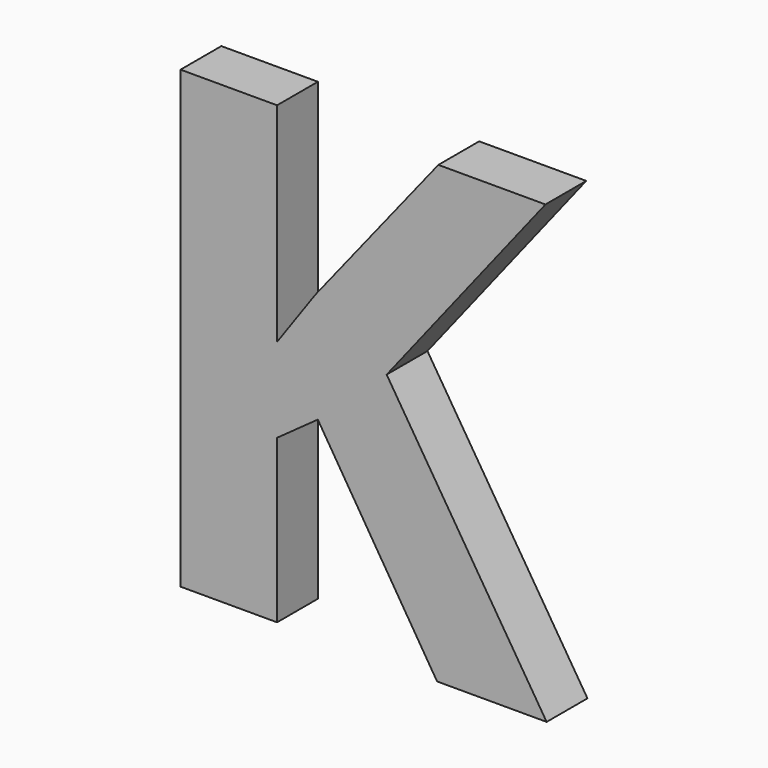
from build123d import *

# Parameters (mm, degrees)
F0_TEXT_SIZE = 62.5
F1_DEPTH     = 5


# Not quite as in the source:
# - Text() gives the source's letters only with a copy of the font that has no kerning and outlines rounded to 1/6400 em; it was checked with that copy


with BuildPart() as f1:
    # F0 (on Front) → F1 (new body)
    with BuildSketch(Plane.XZ):
        with Locations((-63.7499933329, 14.516126955)):
            Text('K', F0_TEXT_SIZE, font='Open Sans', font_style=FontStyle.BOLD, text_align=(TextAlign.LEFT, TextAlign.BOTTOM))
    extrude(amount=F1_DEPTH)


solid = f1.part
